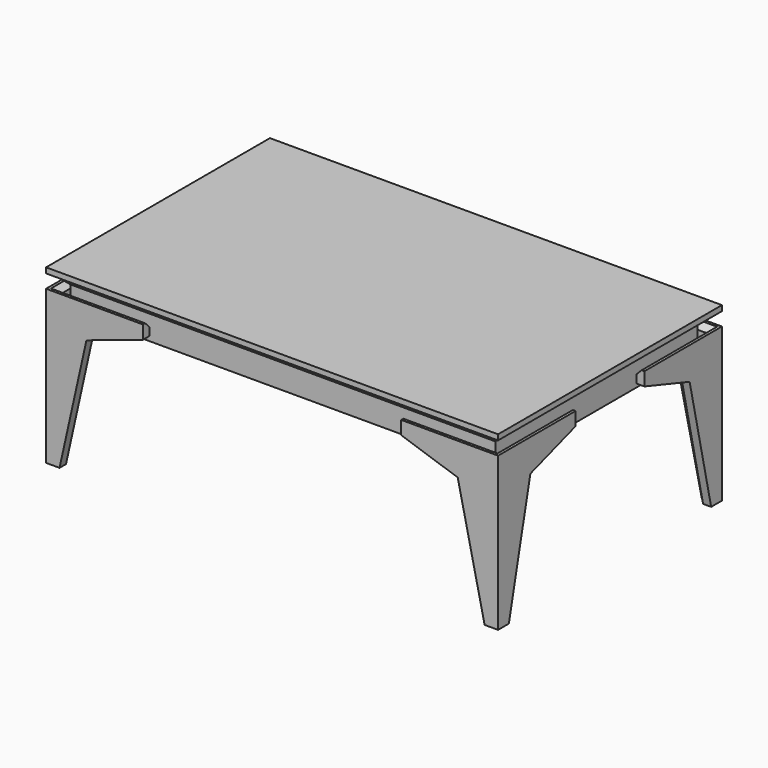
from build123d import *

# Parameters (mm, degrees)
F1_W      = 1066.8
F1_H      = 660.4
F2_DEPTH  = 12.7
F3_W      = 1054.1
F3_H      = 647.7
F4_DEPTH  = 25.4
F4_TAPER  = 45
F6_DEPTH  = 19.05
F7_SIZE   = 12.7
F8_SIZE   = 19.04999
F10_DEPTH = 19.05
F11_SIZE  = 12.7
F12_SIZE  = 19.04999
F15_W     = 1003.3
F15_H     = 596.9
F15_W_2   = 965.2
F15_H_2   = 558.8
F16_DEPTH = 57.15


# Not quite as in the source:
# - a fillet or chamfer is up to 0.001 mm smaller than in the source, because OpenCascade refuses the exact size


with BuildPart() as f2:
    # F1 (on offset) → F2 (new body)
    with BuildSketch(Plane.XY.offset(406.4)):
        Rectangle(F1_W, F1_H)
    extrude(amount=-F2_DEPTH)

    # F3 (on face) → F4 (join)
    with BuildSketch(Plane(origin=(0, 0, 393.7), x_dir=(1, 0, 0), z_dir=(0, 0, -1))):
        Rectangle(F3_W, F3_H)
    extrude(amount=F4_DEPTH, taper=F4_TAPER)


with BuildPart() as f6:
    # F5 (on face) → F6 (new body)
    with BuildSketch(Plane.XZ.offset(330.2)):
        Polygon((-304.8, 361.95), (-533.4, 361.95), (-533.4, 0), (-501.65, 0), (-438.15, 285.75), (-304.8, 330.2), align=None)
    extrude(amount=-F6_DEPTH)

    # F7
    f7_edges = [f6.edges().sort_by_distance(p)[0] for p in [
        (-419.1, -311.15, 361.95),
    ]]
    chamfer(f7_edges, length=F7_SIZE)

    # F8 (size 19.05 in the source; OpenCascade refuses exactly that, so slightly less here)
    f8_edges = [f6.edges().sort_by_distance(p)[0] for p in [
        (-533.4, -311.15, 174.625),
    ]]
    chamfer(f8_edges, length=F8_SIZE)


with BuildPart() as f10:
    # F9 (on face) → F10 (new body)
    with BuildSketch(Plane(origin=(-533.4, 0, 0), x_dir=(0, -1, 0), z_dir=(-1, 0, 0))):
        Polygon((234.95, 285.75), (298.45, 0), (330.2, 0), (330.2, 361.95), (101.6, 361.95), (101.6, 330.2), align=None)
    extrude(amount=-F10_DEPTH)

    # F11
    f11_edges = [f10.edges().sort_by_distance(p)[0] for p in [
        (-514.35, -215.9, 361.95),
    ]]
    chamfer(f11_edges, length=F11_SIZE)

    # F12 (size 19.05 in the source; OpenCascade refuses exactly that, so slightly less here)
    f12_edges = [f10.edges().sort_by_distance(p)[0] for p in [
        (-514.35, -330.2, 174.625),
    ]]
    chamfer(f12_edges, length=F12_SIZE)


with BuildPart() as f13_1:
    # F13: instance of F6
    add(f6.part.mirror(Plane.XZ))


with BuildPart() as f13_2:
    # F13: instance of F10
    add(f10.part.mirror(Plane.XZ))


with BuildPart() as f14_1:
    # F14: instance of F6
    add(f6.part.mirror(Plane.YZ))


with BuildPart() as f14_2:
    # F14: instance of F10
    add(f10.part.mirror(Plane.YZ))


with BuildPart() as f14_3:
    # F14: instance of F13_1
    add(f13_1.part.mirror(Plane.YZ))


with BuildPart() as f14_4:
    # F14: instance of F13_2
    add(f13_2.part.mirror(Plane.YZ))


with BuildPart() as f16:
    # F15 (on face) → F16 (new body)
    with BuildSketch(Plane(origin=(0, 0, 368.3), x_dir=(1, 0, 0), z_dir=(0, 0, -1))):
        Rectangle(F15_W, F15_H)
        Rectangle(F15_W_2, F15_H_2, mode=Mode.SUBTRACT)
    extrude(amount=F16_DEPTH)


solid = Compound([f2.part, f6.part, f10.part, f13_1.part, f13_2.part, f14_1.part, f14_2.part, f14_3.part, f14_4.part, f16.part])
